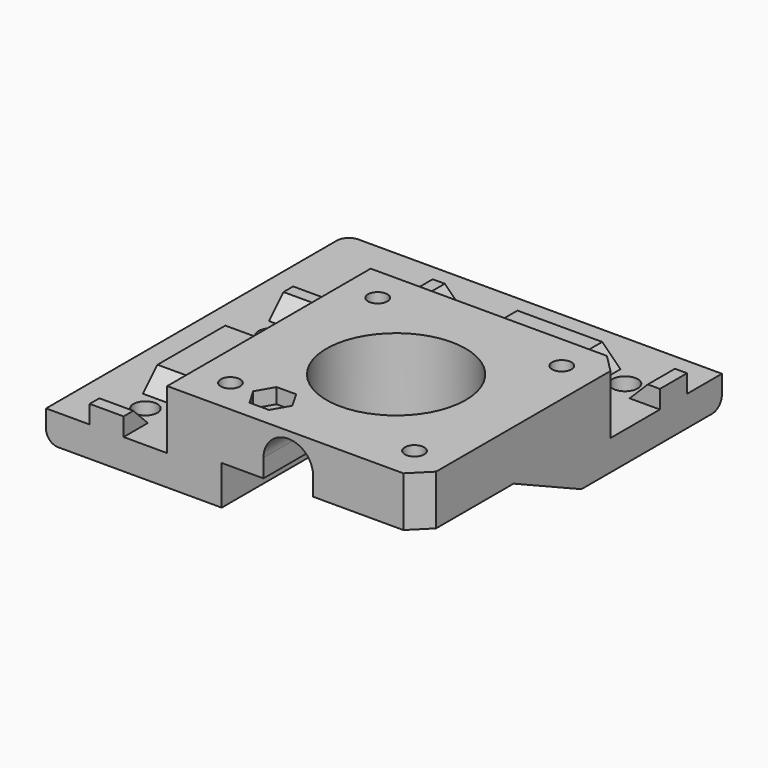
from build123d import *

# Parameters (mm, degrees)
F0_W      = 59
F0_H      = 54
F1_DEPTH  = 5
F2_W      = 42
F2_H      = 42
F3_DEPTH  = 9.75
F5_DEPTH  = 33
F6_R      = 1.6
F6_R_2    = 11.5
F7_DEPTH  = 14.751
F8_SIZE   = 3
F9_R      = 1.6
F10_DEPTH = 2.5
F12_DEPTH = 10.6937211186
F14_DEPTH = 5.001
F16_DEPTH = 20
F18_DEPTH = 20
F19_R     = 2
F20_W     = 5.6
F20_H     = 20
F20_H_2   = 5
F20_W_2   = 5
F20_H_3   = 5.6
F20_W_3   = 20
F21_DEPTH = 3
F22_SIZE  = 2.99999
F23_R     = 1.9824364908
F23_R_2   = 2.1
F24_DEPTH = 5.001


# Not quite as in the source:
# - a fillet or chamfer is up to 0.001 mm smaller than in the source, because OpenCascade refuses the exact size


with BuildPart() as f1:
    # F0 (on Top) → F1 (new body)
    with BuildSketch(Plane.XY):
        with Locations((29.5, 27)):
            Rectangle(F0_W, F0_H)
    extrude(amount=F1_DEPTH)

    # F2 (on face) → F3 (join)
    with BuildSketch(Plane.XY.offset(5)):
        with Locations((38, 21)):
            Rectangle(F2_W, F2_H)
    extrude(amount=F3_DEPTH)

    # F4 (on face) → F5 (cut)
    with BuildSketch(Plane.YZ.offset(59)):
        Polygon((0, 6.5), (0, 0), (33, 0), (19, 6.5), align=None)
    extrude(amount=-F5_DEPTH, mode=Mode.SUBTRACT)

    # F6 (on face) → F7 (cut, through all)
    with BuildSketch(Plane.XY.offset(14.75)):
        with Locations((22.8, 36.2)):
            Circle(F6_R)
        with Locations((38, 21)):
            Circle(F6_R_2)
        with Locations((53.2, 36.2)):
            Circle(F6_R)
        with Locations((22.8, 5.8)):
            Circle(F6_R)
        with Locations((53.2, 5.8)):
            Circle(F6_R)
        with Locations((29.8, 5.8)):
            Circle(F6_R)
    extrude(amount=-F7_DEPTH, mode=Mode.SUBTRACT)

    # F8
    f8_edges = [f1.edges().sort_by_distance(p)[0] for p in [
        (59, 42, 9.875),
        (59, 0, 10.625),
    ]]
    chamfer(f8_edges, length=F8_SIZE)

    # F9 (on face) → F10 (cut)
    with BuildSketch(Plane.XY.offset(14.75)):
        Polygon((31.417729554, 3.0006632601), (33.0331615075, 5.8013265202), (31.4154319535, 8.6006632601), (28.182270446, 8.5993367399), (26.5668384925, 5.7986734798), (28.1845680465, 2.9993367399), align=None)
        with Locations((29.8, 5.8)):
            Circle(F9_R, mode=Mode.SUBTRACT)
    extrude(amount=-F10_DEPTH, mode=Mode.SUBTRACT)

    # F11 (on face) → F12 (cut, through all)
    with BuildSketch(Plane.XZ):
        with BuildLine():
            Line((32.9, 9.5), (32.9, 6.5))
            Line((32.9, 6.5), (41.1, 6.5))
            Line((41.1, 6.5), (41.1, 9.5))
            ThreePointArc((41.1, 9.5), (37, 13.6), (32.9, 9.5))
        make_face()
    extrude(amount=-F12_DEPTH, mode=Mode.SUBTRACT)

    # F13 (on face) → F14 (cut, through all)
    with BuildSketch(Plane.XY.offset(5)):
        Polygon((17, 42), (56, 42), (59, 42), (59, 54), (0, 54), (0, 0), (17, 0), align=None)
    extrude(amount=-F14_DEPTH, mode=Mode.SUBTRACT)

    # F15 (on face) → F16 (join)
    with BuildSketch(Plane(origin=(0, 42, 0), x_dir=(-1, 0, 0), z_dir=(0, 1, 0))):
        Polygon((-56, 5), (-59, 5), (-59, 0), (-17, 0), (-17, 5), align=None)
    extrude(amount=F16_DEPTH)

    # F17 (on face) → F18 (join)
    with BuildSketch(Plane(origin=(17, 0, 0), x_dir=(0, -1, 0), z_dir=(-1, 0, 0))):
        Polygon((-42, 5), (-62, 5), (-62, 0), (0, 0), (0, 5), align=None)
    extrude(amount=F18_DEPTH)

    # F19
    f19_edges = [f1.edges().sort_by_distance(p)[0] for p in [
        (-3, 62, 2.5),
        (-3, 31, 0),
        (28, 62, 0),
    ]]
    fillet(f19_edges, radius=F19_R)

    # F20 (on face) → F21 (join)
    with BuildSketch(Plane.XY.offset(5)):
        with Locations((7, 21)):
            Rectangle(F20_W, F20_H)
        with Locations((7, 39.5)):
            Rectangle(F20_W, F20_H_2)
        with Locations((7, 2.5)):
            Rectangle(F20_W, F20_H_2)
        with Locations((19.5, 52)):
            Rectangle(F20_W_2, F20_H_3)
        with Locations((38, 52)):
            Rectangle(F20_W_3, F20_H_3)
        with Locations((56.5, 52)):
            Rectangle(F20_W_2, F20_H_3)
    extrude(amount=F21_DEPTH)

    # F22 (size 3 in the source; OpenCascade refuses exactly that, so slightly less here)
    f22_edges = [f1.edges().sort_by_distance(p)[0] for p in [
        (54, 52, 8),
        (48, 52, 8),
        (28, 52, 8),
        (22, 52, 8),
        (7, 37, 8),
        (7, 31, 8),
        (7, 11, 8),
        (7, 5, 8),
    ]]
    chamfer(f22_edges, length=F22_SIZE)

    # F23 (on face) → F24 (cut, through all)
    with BuildSketch(Plane.XY.offset(5)):
        with Locations((7, 8)):
            Circle(F23_R)
        with Locations((7, 34)):
            Circle(F23_R_2)
        with Locations((25, 52)):
            Circle(F23_R_2)
        with Locations((51, 52)):
            Circle(F23_R_2)
    extrude(amount=-F24_DEPTH, mode=Mode.SUBTRACT)


solid = f1.part
